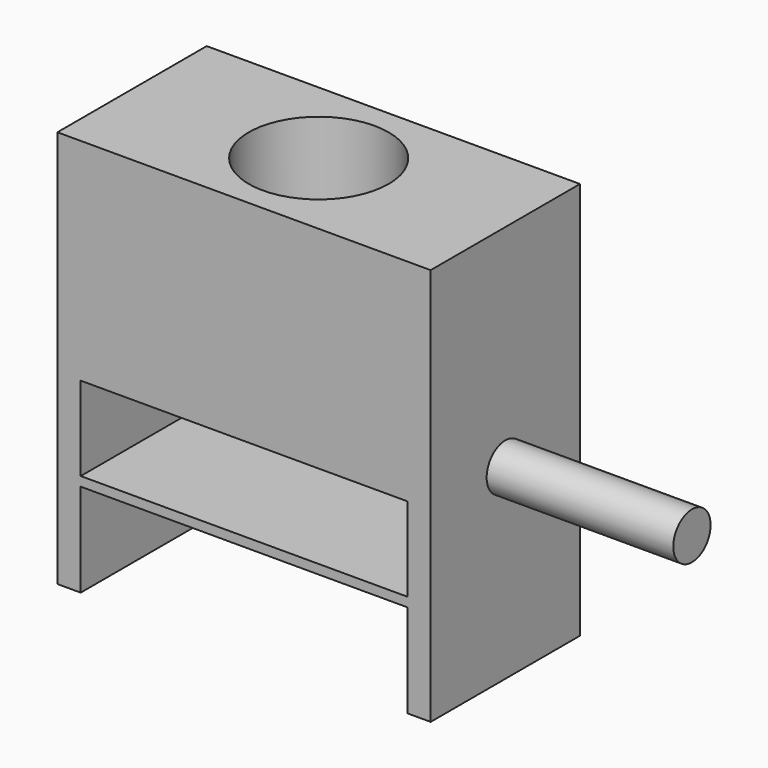
from build123d import *

# Parameters (mm, degrees)
F0_W     = 44.45
F0_H     = 1.27
F1_DEPTH = 25.4
F2_R     = 9.525
F3_DEPTH = 38.1
F4_W     = 1.27
F4_H     = 11.43
F5_DEPTH = 44.45
F6_R     = 3.175
F7_DEPTH = 25.4


with BuildPart() as f1:
    # F0 (on Front) → F1 (new body)
    with BuildSketch(Plane.XZ):
        Polygon((-22.225, -11.43), (-22.225, 0), (-25.4, 0), (-25.4, -25.4), (-22.225, -25.4), (-22.225, -12.7), align=None)
        Polygon((25.4, 0), (22.225, 0), (22.225, -11.43), (22.225, -12.7), (22.225, -25.4), (25.4, -25.4), align=None)
        Polygon((-22.225, 0), (0, 0), (22.225, 0), (25.4, 0), (25.4, 28.7261897342), (-25.4, 28.7261897342), (-25.4, 0), align=None)
        with Locations((0, -12.065)):
            Rectangle(F0_W, F0_H)
    extrude(amount=F1_DEPTH)

    # F2 (on face) → F3 (cut)
    with BuildSketch(Plane.XY.offset(28.7261897342)):
        with Locations((0, -12.7)):
            Circle(F2_R)
    extrude(amount=-F3_DEPTH, mode=Mode.SUBTRACT)

    # F4 (on face) → F5 (join)
    with BuildSketch(Plane.YZ.offset(-22.225)):
        with Locations((-0.635, -5.715)):
            Rectangle(F4_W, F4_H)
    extrude(amount=F5_DEPTH)

    # F6 (on face) → F7 (join)
    with BuildSketch(Plane.YZ.offset(25.4)):
        with Locations((-12.7, 0)):
            Circle(F6_R)
    extrude(amount=F7_DEPTH)


solid = f1.part
